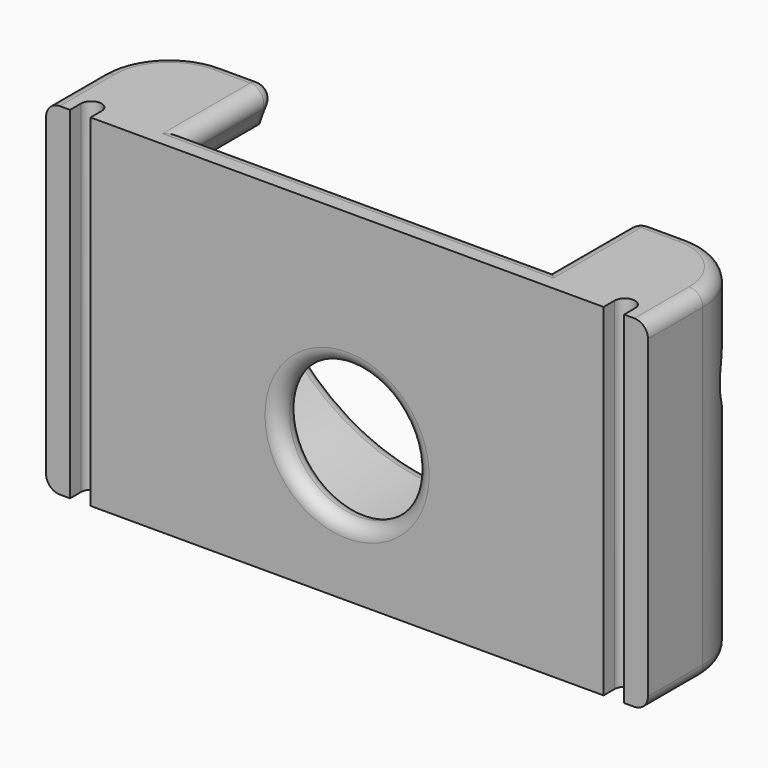
from build123d import *

# Parameters (mm, degrees)
F1_DEPTH    = 25
F2_D        = 4
F2_DEPTH    = 17
F2_TIP      = 1.2017212381
F3_R        = 5
F4_DEPTH    = 10.001
F3_R_2      = 2.075
F5_DEPTH    = 8
F6_T1_DEPTH = 50
F8_DEPTH    = 25.0010001
F9_R        = 0.99999


# Not quite as in the source:
# - a fillet or chamfer that OpenCascade refuses, or shapes differently, is made with other operations: its cross-section is extruded or revolved along the edge and cut away or added
# - a fillet or chamfer is up to 0.001 mm smaller than in the source, because OpenCascade refuses the exact size


with BuildPart() as f1:
    # F0 (on Top) → F1 (new body)
    with BuildSketch(Plane.XY):
        Polygon((22, 10), (0, 10), (-22, 10), (-22, 0), (-17, 0), (0, 0), (17, 0), (22, 0), align=None)
    extrude(amount=F1_DEPTH)

    # F2
    with Locations(Plane(origin=(0, 0, 0), x_dir=(1, 0, 0), z_dir=(0, 0, -1))):
        with Locations((-17, -5), (17, -5)):
            Hole(F2_D / 2, depth=F2_DEPTH)
            with Locations((0, 0, -(F2_DEPTH + F2_TIP / 2))):  # 118° drill point
                Cone(0, F2_D / 2, F2_TIP, mode=Mode.SUBTRACT)

    # F3 (on face) → F4 (cut, through all)
    with BuildSketch(Plane(origin=(0, 10, 0), x_dir=(-1, 0, 0), z_dir=(0, 1, 0))):
        with Locations((0, 10)):
            Circle(F3_R)
    extrude(amount=-F4_DEPTH, mode=Mode.SUBTRACT)

    # F3 (on face) → F5 (cut)
    with BuildSketch(Plane(origin=(0, 10, 0), x_dir=(-1, 0, 0), z_dir=(0, 1, 0))):
        with BuildLine():
            ThreePointArc((13.9373598648, 22), (14.3586510167, 20.0196883375), (14.5, 18))
            ThreePointArc((14.5, 18), (14.3586510167, 15.9803116625), (13.9373598648, 14))
            Line((13.9373598648, 14), (17.5, 14))
            ThreePointArc((17.5, 14), (21.5, 18), (17.5, 22))
            Line((17.5, 22), (13.9373598648, 22))
        make_face()
        with Locations((17.5, 18)):
            Circle(F3_R_2, mode=Mode.SUBTRACT)
        with BuildLine():
            ThreePointArc((13.9373598648, 14), (14.3586510167, 15.9803116625), (14.5, 18))
            ThreePointArc((14.5, 18), (14.3586510167, 20.0196883375), (13.9373598648, 22))
            ThreePointArc((13.9373598648, 22), (13.4020990954, 23.5347755003), (12.6984250992, 25))
            Line((12.6984250992, 25), (-12.6984250992, 25))
            ThreePointArc((-12.6984250992, 25), (-13.4020990954, 23.5347755003), (-13.9373598648, 22))
            ThreePointArc((-13.9373598648, 22), (-14.5, 18), (-13.9373598648, 14))
            ThreePointArc((-13.9373598648, 14), (0, 3.5), (13.9373598648, 14))
        make_face()
        with Locations((0, 10)):
            Circle(F3_R, mode=Mode.SUBTRACT)
        with BuildLine():
            Line((-17.5, 14), (-13.9373598648, 14))
            ThreePointArc((-13.9373598648, 14), (-14.5, 18), (-13.9373598648, 22))
            Line((-13.9373598648, 22), (-17.5, 22))
            ThreePointArc((-17.5, 22), (-21.5, 18), (-17.5, 14))
        make_face()
        with Locations((-17.5, 18)):
            Circle(F3_R_2, mode=Mode.SUBTRACT)
        with Locations((17.5, 18)):
            Circle(F3_R_2)
        with Locations((-17.5, 18)):
            Circle(F3_R_2)
    extrude(amount=-F5_DEPTH, mode=Mode.SUBTRACT)

    # F6: fillet of radius 5 on 2 edges, made by hand

    # F6_s2 → F6_t1 (cut)
    with BuildSketch(Plane.XY.offset(-12.5)):
        with BuildLine():
            ThreePointArc((-17, 10), (-20.5355339059, 8.5355339059), (-22, 5))
            Line((-22, 5), (-22, 10))
            Line((-22, 10), (-17, 10))
        make_face()
        with BuildLine():
            ThreePointArc((17, 10), (20.5355339059, 8.5355339059), (22, 5))
            Line((22, 5), (22, 10))
            Line((22, 10), (17, 10))
        make_face()
    extrude(amount=F6_T1_DEPTH, mode=Mode.SUBTRACT)

    # F7 (on face) → F8 (cut, through all)
    with BuildSketch(Plane.XY.offset(25)):
        with BuildLine():
            ThreePointArc((-18.75, 1), (-19.5, 1.75), (-20.25, 1))
            Line((-20.25, 1), (-18.75, 1))
        make_face()
        with BuildLine():
            Line((-18.75, 1), (-20.25, 1))
            ThreePointArc((-20.25, 1), (-19.5, 0.25), (-18.75, 1))
        make_face()
        with BuildLine():
            Line((-20.25, 1), (-20.25, 0))
            Line((-20.25, 0), (-18.75, 0))
            Line((-18.75, 0), (-18.75, 1))
            ThreePointArc((-18.75, 1), (-19.5, 0.25), (-20.25, 1))
        make_face()
        with BuildLine():
            ThreePointArc((20.25, 1), (19.5, 1.75), (18.75, 1))
            ThreePointArc((18.75, 1), (19.5, 0.25), (20.25, 1))
        make_face()
        with BuildLine():
            Line((18.75, 1), (18.75, 0))
            Line((18.75, 0), (20.25, 0))
            Line((20.25, 0), (20.25, 1))
            ThreePointArc((20.25, 1), (19.5, 0.25), (18.75, 1))
        make_face()
    extrude(amount=-F8_DEPTH, mode=Mode.SUBTRACT)

    # F9 (radius 1 in the source; OpenCascade refuses exactly that, so slightly less here)
    f9_edges = [f1.edges().sort_by_distance(p)[0] for p in [
        (5, 0, 10),
        (5, 2, 10),
        (0, 10, 3.5),
        (13.402099, 10, 23.534776),
        (-13.402099, 10, 23.534776),
        (0, 10, 0),
        (20.535534, 8.535534, 25),
        (-20.535534, 8.535534, 25),
        (13.93736, 6, 22),
        (13.93736, 6, 14),
        (-13.93736, 6, 14),
        (-13.93736, 6, 22),
        (-12.698425, 6, 25),
        (12.698425, 6, 25),
        (0, 2, 25),
        (20.535534, 8.535534, 0),
        (22, 2.5, 0),
        (-22, 2.5, 0),
        (-20.535534, 8.535534, 0),
        (-19, 5, 0),
        (15, 5, 0),
        (22, 2.5, 25),
        (-22, 2.5, 25),
        (-14.849213, 10, 25),
        (14.849213, 10, 25),
    ]]
    fillet(f9_edges, radius=F9_R)


solid = f1.part
